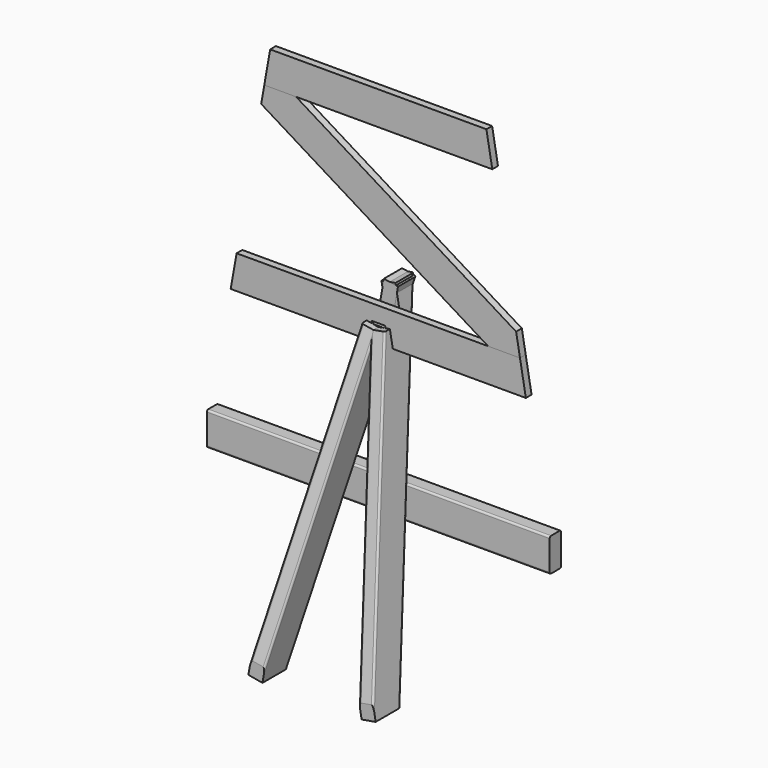
from build123d import *

# Parameters (mm, degrees)
F5_DEPTH      = 38.1
F6_DEPTH      = 38.1
F7_R          = 6.35
F7_2_R        = 6.35
F8_R          = 6.35
F9_DEPTH      = 169.842086772
F9_DEPTH_BACK = 169.842086772
F11_DEPTH     = 19.05
F13_DEPTH     = 19.05
F15_DEPTH     = 19.05
F16_W         = 914.4
F16_H         = 88.9
F17_DEPTH     = 19.05
F18_R         = 4.7752
F18_2_R       = 4.7752
F18_3_R       = 4.7752


with BuildPart() as f5:
    # F3 (on line) → F5 (new body)
    with BuildSketch(Plane(origin=(0, 0, 0), x_dir=(0, 1, 0), z_dir=(0.984807753, 0, 0.1736481777))):
        Polygon((19.05, 38.1), (-35.8091619876, 38.1), (-239.9864466201, -723.9), (-239.9864466201, -762), (-158.1592584133, -762), (80.047573658, 127), (19.05, 127), align=None)
    extrude(amount=F5_DEPTH)

    # F7
    f7_edges = [f5.edges().sort_by_distance(p)[0] for p in [
        (12.144592, 19.05, 40.829173),
    ]]
    fillet(f7_edges, radius=F7_R)


with BuildPart() as f6:
    # F4 (on line) → F6 (new body)
    with BuildSketch(Plane(origin=(0, 0, 0), x_dir=(0, 1, 0), z_dir=(0.984807753, 0, -0.1736481777))):
        Polygon((19.05, 38.1), (-35.8091619876, 38.1), (-239.9864466201, -723.9), (-239.9864466201, -762), (-158.1592584133, -762), (80.047573658, 127), (19.05, 127), align=None)
    extrude(amount=-F6_DEPTH)

    # F7#2
    f7_2_edges = [f6.edges().sort_by_distance(p)[0] for p in [
        (-12.144592, 19.05, 40.829173),
    ]]
    fillet(f7_2_edges, radius=F7_2_R)


with BuildPart() as f9_tool:
    # F8 (on Right) → F9 (new body, two sides)
    with BuildSketch(Plane.YZ) as f9_sk:
        Circle(F8_R)
    extrude(amount=F9_DEPTH)
    extrude(f9_sk.sketch, amount=-F9_DEPTH_BACK)


with BuildPart() as f5_1:
    add(f5.part)

    # F9: cut by f9_tool
    add(f9_tool.part, mode=Mode.SUBTRACT)

    # F18
    f18_edges = [f5_1.edges().sort_by_distance(p)[0] for p in [
        (97.065136, -137.897804, -331.074583),
        (59.54396, -137.897804, -337.690579),
        (92.654472, -39.055842, -306.060466),
        (55.133296, -39.055842, -312.676462),
        (11.041926, 19.05, 47.082702),
    ]]
    fillet(f18_edges, radius=F18_R)


with BuildPart() as f6_1:
    add(f6.part)

    # F9: cut by f9_tool
    add(f9_tool.part, mode=Mode.SUBTRACT)

    # F18#2
    f18_2_edges = [f6_1.edges().sort_by_distance(p)[0] for p in [
        (-59.54396, -137.897804, -337.690579),
        (-55.133296, -39.055842, -312.676462),
        (-97.065136, -137.897804, -331.074583),
        (-92.654472, -39.055842, -306.060466),
    ]]
    fillet(f18_2_edges, radius=F18_2_R)


with BuildPart() as f11:
    # F10 (on Front) → F11 (new body)
    with BuildSketch(Plane.XZ):
        Polygon((378.024531415, 88.9), (-378.024531415, 88.9), (-393.7, 0), (393.7, 0), align=None)
        with BuildLine():
            ThreePointArc((19.05, 44.45), (18.1200640303, 42.2049359697), (15.875, 41.275))
            Line((15.875, 41.275), (-15.875, 41.275))
            ThreePointArc((-15.875, 41.275), (-18.1200640303, 42.2049359697), (-19.05, 44.45))
            ThreePointArc((-19.05, 44.45), (-18.1200640303, 46.6950640303), (-15.875, 47.625))
            Line((-15.875, 47.625), (15.875, 47.625))
            ThreePointArc((15.875, 47.625), (18.1200640303, 46.6950640303), (19.05, 44.45))
        make_face(mode=Mode.SUBTRACT)
    extrude(amount=F11_DEPTH)


with BuildPart() as f13:
    # F12 (on Front) → F13 (new body)
    with BuildSketch(Plane.XZ):
        Polygon((288.4504252151, 596.9), (-288.4504252151, 596.9), (-304.1258938001, 508), (304.1258938001, 508), align=None)
    extrude(amount=F13_DEPTH)


with BuildPart() as f15:
    # F14 (on Front) → F15 (new body)
    with BuildSketch(Plane.XZ):
        Polygon((-219.2128682677, 508), (-304.1258938001, 508), (-312.4255627119, 460.9302385914), (293.1115058827, 88.9), (378.024531415, 88.9), (367.708150879, 147.4071013782), align=None)
    extrude(amount=F15_DEPTH)


with BuildPart() as f17:
    # F16 (on Front) → F17 (new body, symmetric)
    with BuildSketch(Plane.XZ):
        with Locations((0, -349.25)):
            Rectangle(F16_W, F16_H)
    extrude(amount=F17_DEPTH, both=True)

    # F18#3
    f18_3_edges = [f17.edges().sort_by_distance(p)[0] for p in [
        (0, -19.05, -393.7),
        (0, -19.05, -304.8),
        (0, 19.05, -393.7),
        (0, 19.05, -304.8),
    ]]
    fillet(f18_3_edges, radius=F18_3_R)


solid = Compound([f5_1.part, f6_1.part, f11.part, f13.part, f15.part, f17.part])
